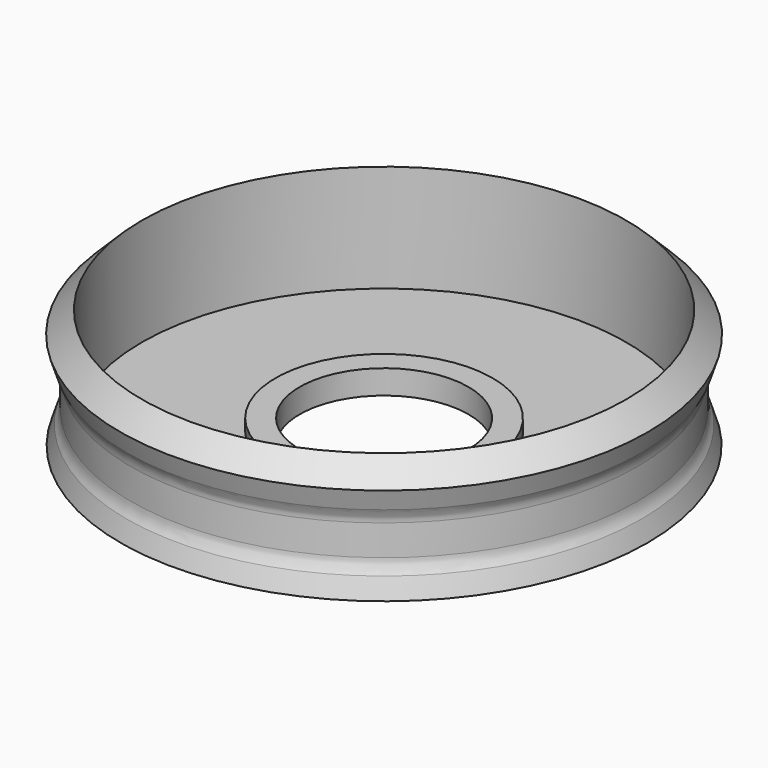
from build123d import *

# Parameters (mm, degrees)
F0_R          = 11
F0_R_2        = 10.5
F0_R_3        = 10.05
F1_DEPTH      = 5
F4_R          = 11
F4_R_2        = 10.5
F5_DEPTH      = 2
F5_DEPTH_BACK = 1
F0_R_4        = 4.5
F9_DEPTH      = 0.5
F0_R_5        = 3.5
F10_DEPTH     = 1


# Not quite as in the source:
# - a fillet or chamfer that OpenCascade refuses, or shapes differently, is made with other operations: its cross-section is extruded or revolved along the edge and cut away or added


with BuildPart() as f1:
    # F0 (on Top) → F1 (new body)
    with BuildSketch(Plane.XY):
        Circle(F0_R)
        Circle(F0_R_2, mode=Mode.SUBTRACT)
        Circle(F0_R_2)
        Circle(F0_R_3, mode=Mode.SUBTRACT)
    extrude(amount=F1_DEPTH)

    # F4 (on plane+point) → F5 (cut, two sides)
    with BuildSketch(Plane.XY.offset(2.5)) as f5_sk:
        Circle(F4_R)
        Circle(F4_R_2, mode=Mode.SUBTRACT)
    extrude(amount=-F5_DEPTH, mode=Mode.SUBTRACT)
    extrude(f5_sk.sketch, amount=F5_DEPTH_BACK, mode=Mode.SUBTRACT)

    # F6: chamfer of 1 on 1 edges, made by hand

    # F6_s1 → F6_t2 (revolve, cut)
    with BuildSketch(Plane.XZ):
        Polygon((11, 4), (10, 5), (11, 5), align=None)
    revolve(axis=Axis((0, 0, 5), (0, 0, 1)), mode=Mode.SUBTRACT)

    # F7: fillet of radius 1 on 2 edges, made by hand

    # F7_s1 → F7_t2 (revolve)
    with BuildSketch(Plane.XZ):
        with BuildLine():
            ThreePointArc((10.5, 2.6339745962), (10.6339745962, 3.1339745962), (11, 3.5))
            Line((11, 3.5), (10.5, 3.5))
            Line((10.5, 3.5), (10.5, 2.6339745962))
        make_face()
    revolve(axis=Axis((0, 0, 3.5), (0, 0, 1)))

    # F7_s3 → F7_t4 (revolve)
    with BuildSketch(Plane.XZ):
        with BuildLine():
            ThreePointArc((11, 0.5), (10.6339745962, 0.8660254038), (10.5, 1.3660254038))
            Line((10.5, 1.3660254038), (10.5, 0.5))
            Line((10.5, 0.5), (11, 0.5))
        make_face()
    revolve(axis=Axis((0, 0, 0.5), (0, 0, 1)))

    # F8: chamfer of 1 on 2 edges, made by hand

    # F8_s1 → F8_t2 (revolve, cut)
    with BuildSketch(Plane.XZ):
        with BuildLine():
            Line((10.6709126952, 3.1725042869), (11.0121000067, 4.2475531418))
            Line((11.0121000067, 4.2475531418), (11.0321000067, 4.2475531418))
            ThreePointArc((11.0321000067, 4.2475531418), (11.02, 3.8737765709), (11.02, 3.5))
            Line((11.02, 3.5), (11.01, 3.4826794919))
            ThreePointArc((11.01, 3.4826794919), (10.8264226951, 3.3457987418), (10.6872524412, 3.1609711736))
            Line((10.6872524412, 3.1609711736), (10.6709126952, 3.1725042869))
        make_face()
    revolve(axis=Axis((0, 0, 3.5), (0, 0, 1)), mode=Mode.SUBTRACT)

    # F8_s3 → F8_t4 (revolve, cut)
    with BuildSketch(Plane.XZ):
        with BuildLine():
            Line((11.0121000067, -0.2475531418), (10.6709126952, 0.8274957131))
            Line((10.6709126952, 0.8274957131), (10.6872524412, 0.8390288264))
            ThreePointArc((10.6872524412, 0.8390288264), (10.8264226951, 0.6542012582), (11.01, 0.5173205081))
            Line((11.01, 0.5173205081), (11.02, 0.5))
            ThreePointArc((11.02, 0.5), (11.02, 0.1262234291), (11.0321000067, -0.2475531418))
            Line((11.0321000067, -0.2475531418), (11.0121000067, -0.2475531418))
        make_face()
    revolve(axis=Axis((0, 0, 0.5), (0, 0, 1)), mode=Mode.SUBTRACT)

    # F0 (on Top) → F9 (join)
    with BuildSketch(Plane.XY):
        Circle(F0_R_3)
        Circle(F0_R_4, mode=Mode.SUBTRACT)
    extrude(amount=F9_DEPTH)

    # F0 (on Top) → F10 (join)
    with BuildSketch(Plane.XY):
        Circle(F0_R_4)
        Circle(F0_R_5, mode=Mode.SUBTRACT)
    extrude(amount=F10_DEPTH)


solid = f1.part
